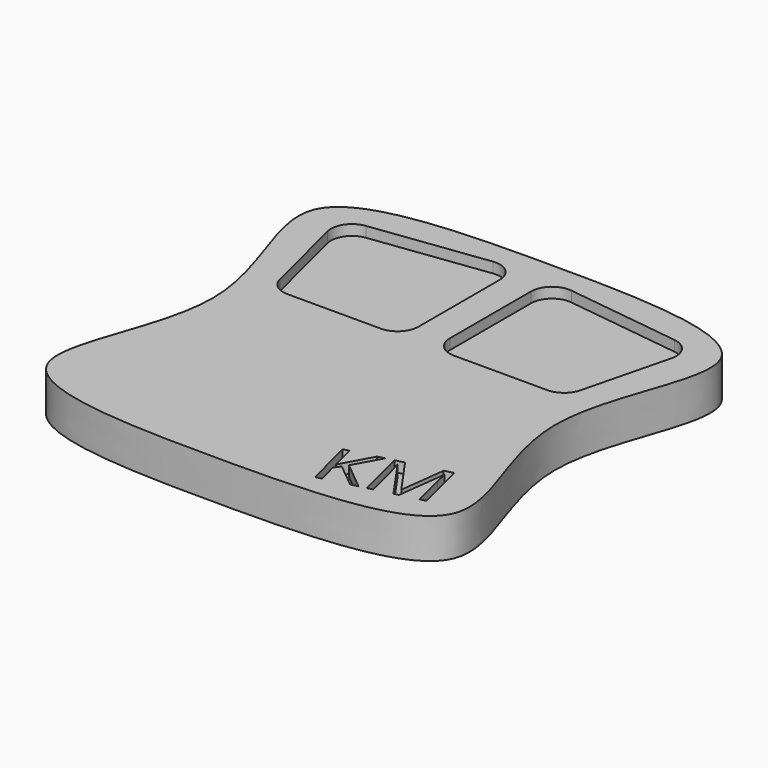
from build123d import *

# Parameters (mm, degrees)
F1_DEPTH     = 19
F2_TEXT_SIZE = 34.7222222222
F3_DEPTH     = 5


# Not quite as in the source:
# - Text() gives the source's letters only with a copy of the font that has no kerning and outlines rounded to 1/6400 em; it was checked with that copy


with BuildPart() as f1:
    # F0 (on Top) → F1 (new body)
    with BuildSketch(Plane.XY):
        with BuildLine():
            add(Edge.make_bspline(
                [(3, 180), (11.161514479, 198.7904164407), (100, 201.2095835593), (229.1066132619, 197.6938721898), (159.6012041815, 100), (229.1066132619, 2.3061278102), (100, -1.2095835593), (-29.1066132619, 2.3061278102), (40.3987958185, 100), (-4.3987958185, 162.9656058385), (3, 180)],
                knots=[0, 0, 0, 0, 0.1311271164, 0.2622542328, 0.3811271164, 0.5, 0.6311271164, 0.7622542328, 0.8811271164, 1, 1, 1, 1], degree=3))
        make_face()
    extrude(amount=F1_DEPTH)

    # F2 (on face) → F3 (cut)
    with BuildSketch(Plane.XY.offset(19)):
        with BuildLine():
            Line((92.5, 130), (92.5, 178.6267744464))
            ThreePointArc((92.5, 178.6267744464), (89.1031381266, 186.1366723739), (81.2202866237, 188.5445531127))
            Line((81.2202866237, 188.5445531127), (26.1478861245, 181.4384369193))
            ThreePointArc((26.1478861245, 181.4384369193), (19.1671760909, 177.1567389026), (17.7261744994, 169.0953020026))
            Line((17.7261744994, 169.0953020026), (28.1063390626, 127.5746437496))
            ThreePointArc((28.1063390626, 127.5746437496), (31.65364197, 122.1179456198), (37.807764064, 120))
            Line((37.807764064, 120), (82.5, 120))
            ThreePointArc((82.5, 120), (89.5710678119, 122.9289321881), (92.5, 130))
        make_face()
        with BuildLine():
            Line((107.5, 178.6267744464), (107.5, 130))
            ThreePointArc((107.5, 130), (110.4289321881, 122.9289321881), (117.5, 120))
            Line((117.5, 120), (162.192235936, 120))
            ThreePointArc((162.192235936, 120), (168.34635803, 122.1179456198), (171.8936609374, 127.5746437496))
            Line((171.8936609374, 127.5746437496), (182.2738255006, 169.0953020026))
            ThreePointArc((182.2738255006, 169.0953020026), (180.8328239091, 177.1567389026), (173.8521138755, 181.4384369193))
            Line((173.8521138755, 181.4384369193), (118.7797133763, 188.5445531127))
            ThreePointArc((118.7797133763, 188.5445531127), (110.8968618734, 186.1366723739), (107.5, 178.6267744464))
        make_face()
        with Locations(Location((135, 10), (0, 0, 13.948234703))):
            Text('KM', F2_TEXT_SIZE, font='Open Sans', text_align=(TextAlign.LEFT, TextAlign.BOTTOM))
    extrude(amount=-F3_DEPTH, mode=Mode.SUBTRACT)


solid = f1.part
